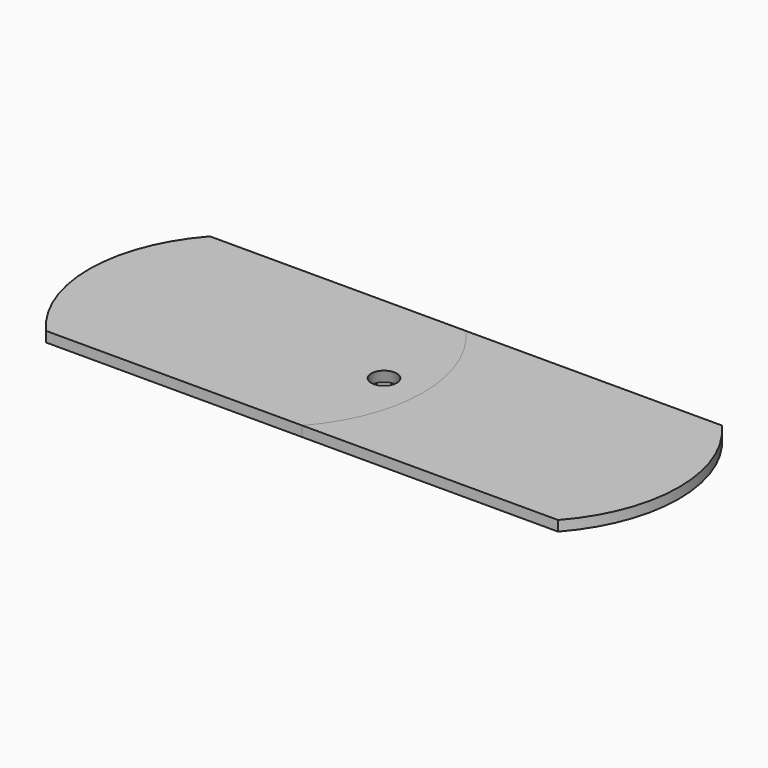
from build123d import *

# Parameters (mm, degrees)
F0_W         = 50
F0_H         = 40
F1_DEPTH     = 2
F2_R         = 2.5
F3_DEPTH     = 25
F4_TEXT_SIZE = 7.3611111111
F5_DEPTH     = 0.5


# Not quite as in the source:
# - Text() gives the source's letters only with a copy of the font that has no kerning and outlines rounded to 1/6400 em; it was checked with that copy


with BuildPart() as f1:
    # F0 (on Top) → F1 (new body)
    with BuildSketch(Plane.XY):
        with BuildLine():
            Line((0, 0), (0, 40))
            ThreePointArc((0, 40), (-7.639320225, 20), (0, 0))
        make_face()
        with BuildLine():
            ThreePointArc((50, 0), (57.639320225, 20), (50, 40))
            Line((50, 40), (50, 0))
        make_face()
        with Locations((25, 20)):
            Rectangle(F0_W, F0_H)
    extrude(amount=F1_DEPTH)

    # F2 (on face) → F3 (cut)
    with BuildSketch(Plane.XY.offset(2)):
        with Locations((0, 20)):
            Circle(F2_R)
    extrude(amount=-F3_DEPTH, mode=Mode.SUBTRACT)

    # F4 (on Top) → F5 (join)
    with BuildSketch(Plane.XY):
        with Locations((2.31627335, 27.7)):
            Text('Michal Duda', F4_TEXT_SIZE, font='Open Sans', font_style=FontStyle.BOLD, text_align=(TextAlign.LEFT, TextAlign.BOTTOM))
        with Locations((2.31627335, 17.6888888889)):
            Text('ur.09.12.2002', F4_TEXT_SIZE, font='Open Sans', font_style=FontStyle.BOLD, text_align=(TextAlign.LEFT, TextAlign.BOTTOM))
        with Locations((2.31627335, 7.6777777778)):
            Text('Grupa krwi : 0', F4_TEXT_SIZE, font='Open Sans', font_style=FontStyle.BOLD, text_align=(TextAlign.LEFT, TextAlign.BOTTOM))
    extrude(amount=-F5_DEPTH)


with BuildPart() as f6_1:
    # F6: instance of F1
    add(f1.part.mirror(Plane.YZ))


solid = Compound([f1.part, f6_1.part])
